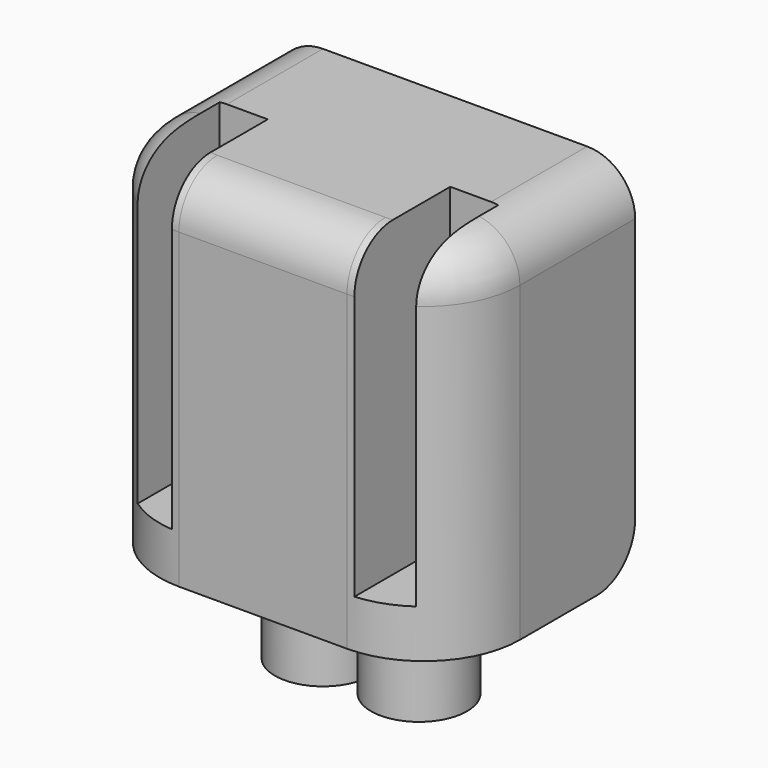
from build123d import *

# Parameters (mm, degrees)
F0_W        = 19.05
F0_H        = 19.05
F1_DEPTH    = 12.7
F2_R        = 2.54
F3_T1_DEPTH = 31.75
F3_T4_ANGLE = 90
F3_T6_ANGLE = 90
F5_W        = 2.54
F5_H        = 16.51
F6_DEPTH    = 6.35
F7_R        = 2.54
F9_DEPTH    = 5.08


# Not quite as in the source:
# - a fillet or chamfer that OpenCascade refuses, or shapes differently, is made with other operations: its cross-section is extruded or revolved along the edge and cut away or added


with BuildPart() as f1:
    # F0 (on Front) → F1 (new body)
    with BuildSketch(Plane.XZ):
        with Locations((0.0981341409, 9.525)):
            Rectangle(F0_W, F0_H)
    extrude(amount=F1_DEPTH)

    # F2
    f2_edges = [f1.edges().sort_by_distance(p)[0] for p in [
        (9.623134, -6.35, 19.05),
        (-9.426866, -6.35, 19.05),
        (0.098134, -12.7, 19.05),
    ]]
    fillet(f2_edges, radius=F2_R)

    # F3: fillet of radius 5.08 on 2 edges, made by hand

    # F3_s2 → F3_t1 (cut)
    with BuildSketch(Plane.XY.offset(-12.7)):
        with BuildLine():
            ThreePointArc((9.6231341409, -7.62), (8.1352365894, -11.2121024484), (4.5431341409, -12.7))
            Line((4.5431341409, -12.7), (9.6231341409, -12.7))
            Line((9.6231341409, -12.7), (9.6231341409, -7.62))
        make_face()
        with BuildLine():
            ThreePointArc((-9.4268658591, -7.62), (-7.9389683075, -11.2121024484), (-4.3468658591, -12.7))
            Line((-4.3468658591, -12.7), (-9.4268658591, -12.7))
            Line((-9.4268658591, -12.7), (-9.4268658591, -7.62))
        make_face()
    extrude(amount=F3_T1_DEPTH, mode=Mode.SUBTRACT)

    # F3_s3 → F3_t4 (revolve, cut)
    with BuildSketch(Plane.XZ.offset(7.62)):
        with BuildLine():
            ThreePointArc((-6.8868658591, 19.05), (-8.6829170833, 18.3060512242), (-9.4268658591, 16.51))
            Line((-9.4268658591, 16.51), (-9.4268658591, 19.05))
            Line((-9.4268658591, 19.05), (-6.8868658591, 19.05))
        make_face()
    revolve(axis=Axis((-4.3468658591, -7.62, 19.05), (0, 0, 1)), revolution_arc=F3_T4_ANGLE, mode=Mode.SUBTRACT)

    # F3_s5 → F3_t6 (revolve, cut)
    with BuildSketch(Plane.YZ.offset(4.5431341409)):
        with BuildLine():
            ThreePointArc((-10.16, 19.05), (-11.9560512242, 18.3060512242), (-12.7, 16.51))
            Line((-12.7, 16.51), (-12.7, 19.05))
            Line((-12.7, 19.05), (-10.16, 19.05))
        make_face()
    revolve(axis=Axis((4.5431341409, -7.62, 19.05), (0, 0, 1)), revolution_arc=F3_T6_ANGLE, mode=Mode.SUBTRACT)

    # F5 (on offset) → F6 (cut)
    with BuildSketch(Plane.XZ.offset(12.7)):
        with Locations((-5.9978658591, 10.795)):
            Rectangle(F5_W, F5_H)
        with Locations((6.1941341409, 10.795)):
            Rectangle(F5_W, F5_H)
    extrude(amount=-F6_DEPTH, mode=Mode.SUBTRACT)

    # F7
    f7_edges = [f1.edges().sort_by_distance(p)[0] for p in [
        (0.098134, 0, 0),
    ]]
    fillet(f7_edges, radius=F7_R)

    # F8 (on face) → F9 (join)
    with BuildSketch(Plane(origin=(0, 0, 0), x_dir=(1, 0, 0), z_dir=(0, 0, -1))):
        with BuildLine():
            ThreePointArc((0.7668002065, 6.7621773998), (0.7035904263, 6.8367161594), (0.6666799214, 6.927209903))
            ThreePointArc((0.6666799214, 6.927209903), (-3.7965534166, 7.9288424314), (-1.8068658591, 3.81))
            Line((-1.8068658591, 3.81), (3.2731341493, 3.81))
            ThreePointArc((3.2731341493, 3.81), (5.2094361027, 7.9938779495), (0.7668002065, 6.7621773998))
        make_face()
    extrude(amount=F9_DEPTH)


solid = f1.part
